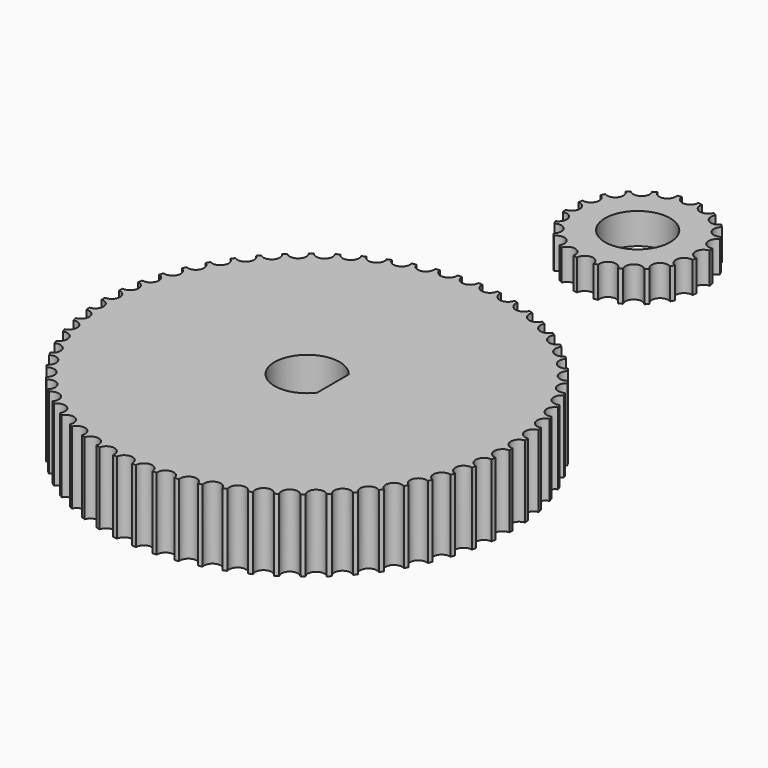
from build123d import *

# Parameters (mm, degrees)
F1_DEPTH = 3
F3_DEPTH = 7


with BuildPart() as f1:
    # F0 (on Top) → F1 (new body)
    with BuildSketch(Plane.XY):
        with BuildLine():
            ThreePointArc((6.3423941927, -0.7984322724), (5.5924532215, 0), (6.3423941927, 0.7984322724))
            ThreePointArc((6.3423941927, 0.7984322724), (6.3137515147, 1), (6.2787044669, 1.2005533751))
            ThreePointArc((6.2787044669, 1.2005533751), (5.3187390784, 1.7281630857), (5.7852461848, 2.7192618061))
            ThreePointArc((5.7852461848, 2.7192618061), (5.6957175259, 2.9021130326), (5.6004114016, 3.0820204934))
            ThreePointArc((5.6004114016, 3.0820204934), (4.5243896964, 3.2871615277), (4.6617979722, 4.3739110479))
            ThreePointArc((4.6617979722, 4.3739110479), (4.5201470213, 4.5201470213), (4.3739110479, 4.6617979722))
            ThreePointArc((4.3739110479, 4.6617979722), (3.2871615277, 4.5243896964), (3.0820204934, 5.6004114016))
            ThreePointArc((3.0820204934, 5.6004114016), (2.9021130326, 5.6957175259), (2.7192618061, 5.7852461848))
            ThreePointArc((2.7192618061, 5.7852461848), (1.7281630857, 5.3187390784), (1.2005533751, 6.2787044669))
            ThreePointArc((1.2005533751, 6.2787044669), (1, 6.3137515147), (0.7984322724, 6.3423941927))
            ThreePointArc((0.7984322724, 6.3423941927), (0, 5.5924532215), (-0.7984322724, 6.3423941927))
            ThreePointArc((-0.7984322724, 6.3423941927), (-1, 6.3137515147), (-1.2005533751, 6.2787044669))
            ThreePointArc((-1.2005533751, 6.2787044669), (-1.1816958118, 6.1799370569), (-1.1753766812, 6.0795842914))
            ThreePointArc((-1.1753766812, 6.0795842914), (-1.825556956, 5.2937382187), (-2.7192618061, 5.7852461848))
            ThreePointArc((-2.7192618061, 5.7852461848), (-2.9021130326, 5.6957175259), (-3.0820204934, 5.6004114016))
            ThreePointArc((-3.0820204934, 5.6004114016), (-2.9891790199, 5.3948795906), (-2.9573897296, 5.1716032919))
            ThreePointArc((-2.9573897296, 5.1716032919), (-3.4864811238, 4.418869257), (-4.3739110479, 4.6617979722))
            ThreePointArc((-4.3739110479, 4.6617979722), (-4.5201470213, 4.5201470213), (-4.6617979722, 4.3739110479))
            ThreePointArc((-4.6617979722, 4.3739110479), (-4.4477786392, 4.0980917579), (-4.3716032919, 3.7573897296))
            ThreePointArc((-4.3716032919, 3.7573897296), (-4.7862764746, 3.0563025425), (-5.6004114016, 3.0820204934))
            ThreePointArc((-5.6004114016, 3.0820204934), (-5.6957175259, 2.9021130326), (-5.7852461848, 2.7192618061))
            ThreePointArc((-5.7852461848, 2.7192618061), (-5.4179686608, 2.4251152245), (-5.2795842914, 1.9753766812))
            ThreePointArc((-5.2795842914, 1.9753766812), (-5.5893272876, 1.3431994353), (-6.2787044669, 1.2005533751))
            ThreePointArc((-6.2787044669, 1.2005533751), (-6.3137515147, 1), (-6.3423941927, 0.7984322724))
            ThreePointArc((-6.3423941927, 0.7984322724), (-5.8093377857, 0.5477010028), (-5.5924532215, 0))
            ThreePointArc((-5.5924532215, 0), (-5.8093377857, -0.5477010028), (-6.3423941927, -0.7984322724))
            ThreePointArc((-6.3423941927, -0.7984322724), (-6.3137515147, -1), (-6.2787044669, -1.2005533751))
            ThreePointArc((-6.2787044669, -1.2005533751), (-5.5893272876, -1.3431994353), (-5.2795842914, -1.9753766812))
            ThreePointArc((-5.2795842914, -1.9753766812), (-5.4179686608, -2.4251152245), (-5.7852461848, -2.7192618061))
            ThreePointArc((-5.7852461848, -2.7192618061), (-5.6957175259, -2.9021130326), (-5.6004114016, -3.0820204934))
            ThreePointArc((-5.6004114016, -3.0820204934), (-4.7862764746, -3.0563025425), (-4.3716032919, -3.7573897296))
            ThreePointArc((-4.3716032919, -3.7573897296), (-4.4477786392, -4.0980917579), (-4.6617979722, -4.3739110479))
            ThreePointArc((-4.6617979722, -4.3739110479), (-4.5201470213, -4.5201470213), (-4.3739110479, -4.6617979722))
            ThreePointArc((-4.3739110479, -4.6617979722), (-3.4864811238, -4.418869257), (-2.9573897296, -5.1716032919))
            ThreePointArc((-2.9573897296, -5.1716032919), (-2.9891790199, -5.3948795906), (-3.0820204934, -5.6004114016))
            ThreePointArc((-3.0820204934, -5.6004114016), (-2.9021130326, -5.6957175259), (-2.7192618061, -5.7852461848))
            ThreePointArc((-2.7192618061, -5.7852461848), (-1.825556956, -5.2937382187), (-1.1753766812, -6.0795842914))
            ThreePointArc((-1.1753766812, -6.0795842914), (-1.1816958118, -6.1799370569), (-1.2005533751, -6.2787044669))
            ThreePointArc((-1.2005533751, -6.2787044669), (-1, -6.3137515147), (-0.7984322724, -6.3423941927))
            ThreePointArc((-0.7984322724, -6.3423941927), (0, -5.5924532215), (0.7984322724, -6.3423941927))
            ThreePointArc((0.7984322724, -6.3423941927), (1, -6.3137515147), (1.2005533751, -6.2787044669))
            ThreePointArc((1.2005533751, -6.2787044669), (1.7281630857, -5.3187390784), (2.7192618061, -5.7852461848))
            ThreePointArc((2.7192618061, -5.7852461848), (2.9021130326, -5.6957175259), (3.0820204934, -5.6004114016))
            ThreePointArc((3.0820204934, -5.6004114016), (3.2871615277, -4.5243896964), (4.3739110479, -4.6617979722))
            ThreePointArc((4.3739110479, -4.6617979722), (4.5201470213, -4.5201470213), (4.6617979722, -4.3739110479))
            ThreePointArc((4.6617979722, -4.3739110479), (4.5243896964, -3.2871615277), (5.6004114016, -3.0820204934))
            ThreePointArc((5.6004114016, -3.0820204934), (5.6957175259, -2.9021130326), (5.7852461848, -2.7192618061))
            ThreePointArc((5.7852461848, -2.7192618061), (5.3187390784, -1.7281630857), (6.2787044669, -1.2005533751))
            ThreePointArc((6.2787044669, -1.2005533751), (6.3137515147, -1), (6.3423941927, -0.7984322724))
        make_face()
        with BuildLine():
            ThreePointArc((2.5, 1.9163767897), (2.9830772702, 1.0118053172), (3.15, 0))
            ThreePointArc((3.15, 0), (2.9830772702, -1.0118053172), (2.5, -1.9163767897))
            ThreePointArc((2.5, -1.9163767897), (-3.15, 0), (2.5, 1.9163767897))
        make_face(mode=Mode.SUBTRACT)
    extrude(amount=F1_DEPTH)


with BuildPart() as f3:
    # F2 (on Top) → F3 (new body)
    with BuildSketch(Plane.XY):
        with BuildLine():
            ThreePointArc((19.7426438555, -40.2003698738), (19.7434064237, -40.1001862267), (19.7436606153, -40))
            ThreePointArc((19.7436606153, -40), (19.7434064237, -39.8998137733), (19.7426438555, -39.7996301262))
            ThreePointArc((19.7426438555, -39.7996301262), (18.9193465628, -39.0405193351), (19.6616218184, -38.2020116903))
            ThreePointArc((19.6616218184, -38.2020116903), (19.6423622777, -38.0025669857), (19.6210796506, -37.8033280088))
            ThreePointArc((19.6210796506, -37.8033280088), (18.7252084651, -37.1314035752), (19.3788449351, -36.2221032999))
            ThreePointArc((19.3788449351, -36.2221032999), (19.3395067226, -36.025630337), (19.2981766169, -35.8295667186))
            ThreePointArc((19.2981766169, -35.8295667186), (18.3389243893, -35.2517234965), (18.8972148789, -34.280961242))
            ThreePointArc((18.8972148789, -34.280961242), (18.8382016581, -34.0894760993), (18.7772481765, -33.8985997173))
            ThreePointArc((18.7772481765, -33.8985997173), (17.7644581327, -33.4207671602), (18.221673826, -32.3985042609))
            ThreePointArc((18.221673826, -32.3985042609), (18.1435911524, -32.213971835), (18.0636397602, -32.0302413394))
            ThreePointArc((18.0636397602, -32.0302413394), (17.0077044965, -31.6573226559), (17.3591537418, -30.5940489125))
            ThreePointArc((17.3591537418, -30.5940489125), (17.2628028493, -30.4183627558), (17.1646739559, -30.2436634703))
            ThreePointArc((17.1646739559, -30.2436634703), (16.0764287971, -29.9794853106), (16.3185052495, -28.8861113505))
            ThreePointArc((16.3185052495, -28.8861113505), (16.2048748287, -28.7210742408), (16.0895753693, -28.5571988163))
            ThreePointArc((16.0895753693, -28.5571988163), (14.9801871834, -28.404472006), (15.110406811, -27.2922173256))
            ThreePointArc((15.110406811, -27.2922173256), (14.9806628636, -27.139522767), (14.8493759667, -26.9881527871))
            ThreePointArc((14.8493759667, -26.9881527871), (13.7302285777, -26.9484445098), (13.7472551508, -25.8287223473))
            ThreePointArc((13.7472551508, -25.8287223473), (13.6027290254, -25.6899371925), (13.4568018723, -25.5526259181))
            ThreePointArc((13.4568018723, -25.5526259181), (12.3393792469, -25.6263436346), (12.2430380499, -24.5106438545))
            ThreePointArc((12.2430380499, -24.5106438545), (12.08521278, -24.3871922271), (11.9261427807, -24.2653486576))
            ThreePointArc((11.9261427807, -24.2653486576), (10.8219111871, -24.4517359243), (10.613190811, -23.3515071162))
            ThreePointArc((10.613190811, -23.3515071162), (10.4436858976, -23.2446557969), (10.2731053255, -23.1395302123))
            ThreePointArc((10.2731053255, -23.1395302123), (9.1933956741, -23.4366744436), (8.8744378725, -22.3632064439))
            ThreePointArc((8.8744378725, -22.3632064439), (8.6949926653, -22.2740518718), (8.514651908, -22.1867230028))
            ThreePointArc((8.514651908, -22.1867230028), (7.4705434809, -22.5915750969), (7.0446211924, -21.5558831399))
            ThreePointArc((7.0446211924, -21.5558831399), (6.8570770421, -21.4853401616), (6.6688266397, -21.4167041206))
            ThreePointArc((6.6688266397, -21.4167041206), (5.6710334024, -21.925109747), (5.142517166, -20.9378214338))
            ThreePointArc((5.142517166, -20.9378214338), (4.9487985293, -20.8866139156), (4.7545701858, -20.8373750013))
            ThreePointArc((4.7545701858, -20.8373750013), (3.8133308469, -21.4441172304), (3.1876439545, -20.515363475))
            ThreePointArc((3.1876439545, -20.515363475), (2.9897386468, -20.4840168755), (2.7915254077, -20.4546803456))
            ThreePointArc((2.7915254077, -20.4546803456), (1.9164983568, -21.1535331811), (1.2000612024, -20.2928442538))
            ThreePointArc((1.2000612024, -20.2928442538), (1, -20.2816802315), (0.7998358015, -20.2725471187))
            ThreePointArc((0.7998358015, -20.2725471187), (0, -21.0563393847), (-0.7998358015, -20.2725471187))
            ThreePointArc((-0.7998358015, -20.2725471187), (-1, -20.2816802315), (-1.2000612024, -20.2928442538))
            ThreePointArc((-1.2000612024, -20.2928442538), (-1.1980903314, -20.3252143475), (-1.1974330143, -20.3576377223))
            ThreePointArc((-1.1974330143, -20.3576377223), (-1.9488218774, -21.1561594549), (-2.7915254077, -20.4546803456))
            ThreePointArc((-2.7915254077, -20.4546803456), (-2.9897386468, -20.4840168755), (-3.1876439545, -20.515363475))
            ThreePointArc((-3.1876439545, -20.515363475), (-3.1776951476, -20.5876254752), (-3.174369663, -20.6604932774))
            ThreePointArc((-3.174369663, -20.6604932774), (-3.885376456, -21.4555279993), (-4.7545701858, -20.8373750013))
            ThreePointArc((-4.7545701858, -20.8373750013), (-4.9487985293, -20.8866139156), (-5.142517166, -20.9378214338))
            ThreePointArc((-5.142517166, -20.9378214338), (-5.118562605, -21.048673163), (-5.1105239007, -21.1617983419))
            ThreePointArc((-5.1105239007, -21.1617983419), (-5.781377068, -21.9513052105), (-6.6688266397, -21.4167041206))
            ThreePointArc((-6.6688266397, -21.4167041206), (-6.8570770421, -21.4853401616), (-7.0446211924, -21.5558831399))
            ThreePointArc((-7.0446211924, -21.5558831399), (-7.0008130422, -21.7033166827), (-6.986028165, -21.8564088476))
            ThreePointArc((-6.986028165, -21.8564088476), (-7.6170592247, -22.63836121), (-8.514651908, -22.1867230028))
            ThreePointArc((-8.514651908, -22.1867230028), (-8.6949926653, -22.2740518718), (-8.8744378725, -22.3632064439))
            ThreePointArc((-8.8744378725, -22.3632064439), (-8.8051839303, -22.5445309851), (-8.7816372442, -22.7371971507))
            ThreePointArc((-8.7816372442, -22.7371971507), (-9.373279937, -23.5095877465), (-10.2731053255, -23.1395302123))
            ThreePointArc((-10.2731053255, -23.1395302123), (-10.4436858976, -23.2446557969), (-10.613190811, -23.3515071162))
            ThreePointArc((-10.613190811, -23.3515071162), (-10.5132273987, -23.5633795764), (-10.4789257592, -23.7951251713))
            ThreePointArc((-10.4789257592, -23.7951251713), (-11.0317149354, -24.555971285), (-11.9261427807, -24.2653486576))
            ThreePointArc((-11.9261427807, -24.2653486576), (-12.08521278, -24.3871922271), (-12.2430380499, -24.5106438545))
            ThreePointArc((-12.2430380499, -24.5106438545), (-12.1074993627, -24.7491069998), (-12.060477233, -25.0193371364))
            ThreePointArc((-12.060477233, -25.0193371364), (-12.5750474793, -25.7666856868), (-13.4568018723, -25.5526259181))
            ThreePointArc((-13.4568018723, -25.5526259181), (-13.6027290254, -25.6899371925), (-13.7472551508, -25.8287223473))
            ThreePointArc((-13.7472551508, -25.8287223473), (-13.5717383106, -26.0892499731), (-13.5100628075, -26.3972709746))
            ThreePointArc((-13.5100628075, -26.3972709746), (-13.9871468179, -27.1292035286), (-14.8493759667, -26.9881527871))
            ThreePointArc((-14.8493759667, -26.9881527871), (-14.9806628636, -27.139522767), (-15.110406811, -27.2922173256))
            ThreePointArc((-15.110406811, -27.2922173256), (-14.891031918, -27.5697660392), (-14.8128077729, -27.91478722))
            ThreePointArc((-14.8128077729, -27.91478722), (-15.2532344682, -28.6294249174), (-16.0895753693, -28.5571988163))
            ThreePointArc((-16.0895753693, -28.5571988163), (-16.2048748287, -28.7210742408), (-16.3185052495, -28.8861113505))
            ThreePointArc((-16.3185052495, -28.8861113505), (-16.0519697783, -29.1751784066), (-15.9553442031, -29.5563141024))
            ThreePointArc((-15.9553442031, -29.5563141024), (-16.3600366028, -30.2518224784), (-17.1646739559, -30.2436634703))
            ThreePointArc((-17.1646739559, -30.2436634703), (-17.2628028493, -30.4183627558), (-17.3591537418, -30.5940489125))
            ThreePointArc((-17.3591537418, -30.5940489125), (-17.0427806856, -30.8887354939), (-16.9259481282, -31.3050073347))
            ThreePointArc((-16.9259481282, -31.3050073347), (-17.2959209811, -31.9796010293), (-18.0636397602, -32.0302413394))
            ThreePointArc((-18.0636397602, -32.0302413394), (-18.1435911524, -32.213971835), (-18.221673826, -32.3985042609))
            ThreePointArc((-18.221673826, -32.3985042609), (-17.8534530591, -32.6925835359), (-17.7146598384, -33.1429229579))
            ThreePointArc((-17.7146598384, -33.1429229579), (-18.0510170182, -33.7948702988), (-18.7772481765, -33.8985997173))
            ThreePointArc((-18.7772481765, -33.8985997173), (-18.8382016581, -34.0894760993), (-18.8972148789, -34.280961242))
            ThreePointArc((-18.8972148789, -34.280961242), (-18.4758372767, -34.5679504823), (-18.3133860844, -35.0512014707))
            ThreePointArc((-18.3133860844, -35.0512014707), (-18.6173177554, -35.6788289184), (-19.2981766169, -35.8295667186))
            ThreePointArc((-19.2981766169, -35.8295667186), (-19.3395067226, -36.025630337), (-19.3788449351, -36.2221032999))
            ThreePointArc((-19.3788449351, -36.2221032999), (-18.9037288671, -36.4953392968), (-18.7159831245, -37.0102613532))
            ThreePointArc((-18.7159831245, -37.0102613532), (-18.9887626872, -37.611957797), (-19.6210796506, -37.8033280088))
            ThreePointArc((-19.6210796506, -37.8033280088), (-19.6423622777, -38.0025669857), (-19.6616218184, -38.2020116903))
            ThreePointArc((-19.6616218184, -38.2020116903), (-19.1329317092, -38.4547286731), (-18.9183197685, -39))
            ThreePointArc((-18.9183197685, -39), (-19.16130059, -39.5742208937), (-19.7426438555, -39.7996301262))
            ThreePointArc((-19.7426438555, -39.7996301262), (-19.7436606153, -40), (-19.7426438555, -40.2003698738))
            ThreePointArc((-19.7426438555, -40.2003698738), (-19.16130059, -40.4257791063), (-18.9183197685, -41))
            ThreePointArc((-18.9183197685, -41), (-19.1329317092, -41.5452713269), (-19.6616218184, -41.7979883097))
            ThreePointArc((-19.6616218184, -41.7979883097), (-19.6423622777, -41.9974330143), (-19.6210796506, -42.1966719912))
            ThreePointArc((-19.6210796506, -42.1966719912), (-18.9887626872, -42.388042203), (-18.7159831245, -42.9897386468))
            ThreePointArc((-18.7159831245, -42.9897386468), (-18.9037288671, -43.5046607032), (-19.3788449351, -43.7778967001))
            ThreePointArc((-19.3788449351, -43.7778967001), (-19.3395067226, -43.974369663), (-19.2981766169, -44.1704332814))
            ThreePointArc((-19.2981766169, -44.1704332814), (-18.6173177554, -44.3211710816), (-18.3133860844, -44.9487985293))
            ThreePointArc((-18.3133860844, -44.9487985293), (-18.4758372767, -45.4320495177), (-18.8972148789, -45.719038758))
            ThreePointArc((-18.8972148789, -45.719038758), (-18.8382016581, -45.9105239007), (-18.7772481765, -46.1014002827))
            ThreePointArc((-18.7772481765, -46.1014002827), (-18.0510170182, -46.2051297012), (-17.7146598384, -46.8570770421))
            ThreePointArc((-17.7146598384, -46.8570770421), (-17.8534530591, -47.3074164641), (-18.221673826, -47.6014957391))
            ThreePointArc((-18.221673826, -47.6014957391), (-18.1435911524, -47.786028165), (-18.0636397602, -47.9697586606))
            ThreePointArc((-18.0636397602, -47.9697586606), (-17.2959209811, -48.0203989707), (-16.9259481282, -48.6949926653))
            ThreePointArc((-16.9259481282, -48.6949926653), (-17.0427806856, -49.1112645061), (-17.3591537418, -49.4059510875))
            ThreePointArc((-17.3591537418, -49.4059510875), (-17.2628028493, -49.5816372442), (-17.1646739559, -49.7563365297))
            ThreePointArc((-17.1646739559, -49.7563365297), (-16.3600366028, -49.7481775216), (-15.9553442031, -50.4436858976))
            ThreePointArc((-15.9553442031, -50.4436858976), (-16.0519697783, -50.8248215934), (-16.3185052495, -51.1138886495))
            ThreePointArc((-16.3185052495, -51.1138886495), (-16.2048748287, -51.2789257592), (-16.0895753693, -51.4428011837))
            ThreePointArc((-16.0895753693, -51.4428011837), (-15.2532344682, -51.3705750826), (-14.8128077729, -52.08521278))
            ThreePointArc((-14.8128077729, -52.08521278), (-14.891031918, -52.4302339608), (-15.110406811, -52.7077826744))
            ThreePointArc((-15.110406811, -52.7077826744), (-14.9806628636, -52.860477233), (-14.8493759667, -53.0118472129))
            ThreePointArc((-14.8493759667, -53.0118472129), (-13.9871468179, -52.8707964714), (-13.5100628075, -53.6027290254))
            ThreePointArc((-13.5100628075, -53.6027290254), (-13.5717383106, -53.9107500269), (-13.7472551508, -54.1712776527))
            ThreePointArc((-13.7472551508, -54.1712776527), (-13.6027290254, -54.3100628075), (-13.4568018723, -54.4473740819))
            ThreePointArc((-13.4568018723, -54.4473740819), (-12.5750474793, -54.2333143132), (-12.060477233, -54.9806628636))
            ThreePointArc((-12.060477233, -54.9806628636), (-12.1074993627, -55.2508930002), (-12.2430380499, -55.4893561455))
            ThreePointArc((-12.2430380499, -55.4893561455), (-12.08521278, -55.6128077729), (-11.9261427807, -55.7346513424))
            ThreePointArc((-11.9261427807, -55.7346513424), (-11.0317149354, -55.444028715), (-10.4789257592, -56.2048748287))
            ThreePointArc((-10.4789257592, -56.2048748287), (-10.5132273987, -56.4366204236), (-10.613190811, -56.6484928838))
            ThreePointArc((-10.613190811, -56.6484928838), (-10.4436858976, -56.7553442031), (-10.2731053255, -56.8604697877))
            ThreePointArc((-10.2731053255, -56.8604697877), (-9.373279937, -56.4904122535), (-8.7816372442, -57.2628028493))
            ThreePointArc((-8.7816372442, -57.2628028493), (-8.8051839303, -57.4554690149), (-8.8744378725, -57.6367935561))
            ThreePointArc((-8.8744378725, -57.6367935561), (-8.6949926653, -57.7259481282), (-8.514651908, -57.8132769972))
            ThreePointArc((-8.514651908, -57.8132769972), (-7.6170592247, -57.36163879), (-6.986028165, -58.1435911524))
            ThreePointArc((-6.986028165, -58.1435911524), (-7.0008130422, -58.2966833173), (-7.0446211924, -58.4441168601))
            ThreePointArc((-7.0446211924, -58.4441168601), (-6.8570770421, -58.5146598384), (-6.6688266397, -58.5832958794))
            ThreePointArc((-6.6688266397, -58.5832958794), (-5.781377068, -58.0486947895), (-5.1105239007, -58.8382016581))
            ThreePointArc((-5.1105239007, -58.8382016581), (-5.118562605, -58.951326837), (-5.142517166, -59.0621785662))
            ThreePointArc((-5.142517166, -59.0621785662), (-4.9487985293, -59.1133860844), (-4.7545701858, -59.1626249987))
            ThreePointArc((-4.7545701858, -59.1626249987), (-3.885376456, -58.5444720007), (-3.174369663, -59.3395067226))
            ThreePointArc((-3.174369663, -59.3395067226), (-3.1776951476, -59.4123745248), (-3.1876439545, -59.484636525))
            ThreePointArc((-3.1876439545, -59.484636525), (-2.9897386468, -59.5159831245), (-2.7915254077, -59.5453196544))
            ThreePointArc((-2.7915254077, -59.5453196544), (-1.9488218774, -58.8438405451), (-1.1974330143, -59.6423622777))
            ThreePointArc((-1.1974330143, -59.6423622777), (-1.1980903314, -59.6747856525), (-1.2000612024, -59.7071557462))
            ThreePointArc((-1.2000612024, -59.7071557462), (-1, -59.7183197685), (-0.7998358015, -59.7274528813))
            ThreePointArc((-0.7998358015, -59.7274528813), (0, -58.9436606153), (0.7998358015, -59.7274528813))
            ThreePointArc((0.7998358015, -59.7274528813), (1, -59.7183197685), (1.2000612024, -59.7071557462))
            ThreePointArc((1.2000612024, -59.7071557462), (1.9164983568, -58.8464668189), (2.7915254077, -59.5453196544))
            ThreePointArc((2.7915254077, -59.5453196544), (2.9897386468, -59.5159831245), (3.1876439545, -59.484636525))
            ThreePointArc((3.1876439545, -59.484636525), (3.8133308469, -58.5558827696), (4.7545701858, -59.1626249987))
            ThreePointArc((4.7545701858, -59.1626249987), (4.9487985293, -59.1133860844), (5.142517166, -59.0621785662))
            ThreePointArc((5.142517166, -59.0621785662), (5.6710334024, -58.074890253), (6.6688266397, -58.5832958794))
            ThreePointArc((6.6688266397, -58.5832958794), (6.8570770421, -58.5146598384), (7.0446211924, -58.4441168601))
            ThreePointArc((7.0446211924, -58.4441168601), (7.4705434809, -57.4084249031), (8.514651908, -57.8132769972))
            ThreePointArc((8.514651908, -57.8132769972), (8.6949926653, -57.7259481282), (8.8744378725, -57.6367935561))
            ThreePointArc((8.8744378725, -57.6367935561), (9.1933956741, -56.5633255564), (10.2731053255, -56.8604697877))
            ThreePointArc((10.2731053255, -56.8604697877), (10.4436858976, -56.7553442031), (10.613190811, -56.6484928838))
            ThreePointArc((10.613190811, -56.6484928838), (10.8219111871, -55.5482640757), (11.9261427807, -55.7346513424))
            ThreePointArc((11.9261427807, -55.7346513424), (12.08521278, -55.6128077729), (12.2430380499, -55.4893561455))
            ThreePointArc((12.2430380499, -55.4893561455), (12.3393792469, -54.3736563654), (13.4568018723, -54.4473740819))
            ThreePointArc((13.4568018723, -54.4473740819), (13.6027290254, -54.3100628075), (13.7472551508, -54.1712776527))
            ThreePointArc((13.7472551508, -54.1712776527), (13.7302285777, -53.0515554902), (14.8493759667, -53.0118472129))
            ThreePointArc((14.8493759667, -53.0118472129), (14.9806628636, -52.860477233), (15.110406811, -52.7077826744))
            ThreePointArc((15.110406811, -52.7077826744), (14.9801871834, -51.595527994), (16.0895753693, -51.4428011837))
            ThreePointArc((16.0895753693, -51.4428011837), (16.2048748287, -51.2789257592), (16.3185052495, -51.1138886495))
            ThreePointArc((16.3185052495, -51.1138886495), (16.0764287971, -50.0205146894), (17.1646739559, -49.7563365297))
            ThreePointArc((17.1646739559, -49.7563365297), (17.2628028493, -49.5816372442), (17.3591537418, -49.4059510875))
            ThreePointArc((17.3591537418, -49.4059510875), (17.0077044965, -48.3426773441), (18.0636397602, -47.9697586606))
            ThreePointArc((18.0636397602, -47.9697586606), (18.1435911524, -47.786028165), (18.221673826, -47.6014957391))
            ThreePointArc((18.221673826, -47.6014957391), (17.7644581327, -46.5792328398), (18.7772481765, -46.1014002827))
            ThreePointArc((18.7772481765, -46.1014002827), (18.8382016581, -45.9105239007), (18.8972148789, -45.719038758))
            ThreePointArc((18.8972148789, -45.719038758), (18.3389243893, -44.7482765035), (19.2981766169, -44.1704332814))
            ThreePointArc((19.2981766169, -44.1704332814), (19.3395067226, -43.974369663), (19.3788449351, -43.7778967001))
            ThreePointArc((19.3788449351, -43.7778967001), (18.7252084651, -42.8685964248), (19.6210796506, -42.1966719912))
            ThreePointArc((19.6210796506, -42.1966719912), (19.6423622777, -41.9974330143), (19.6616218184, -41.7979883097))
            ThreePointArc((19.6616218184, -41.7979883097), (18.9193465628, -40.9594806649), (19.7426438555, -40.2003698738))
        make_face()
        with BuildLine():
            ThreePointArc((2.5, -38.0836232103), (2.9830772702, -38.9881946828), (3.15, -40))
            ThreePointArc((3.15, -40), (2.9830772702, -41.0118053172), (2.5, -41.9163767897))
            ThreePointArc((2.5, -41.9163767897), (-3.15, -40), (2.5, -38.0836232103))
        make_face(mode=Mode.SUBTRACT)
        with BuildLine():
            ThreePointArc((2.5, -41.9163767897), (2.9830772702, -41.0118053172), (3.15, -40))
            ThreePointArc((3.15, -40), (2.9830772702, -38.9881946828), (2.5, -38.0836232103))
            Line((2.5, -38.0836232103), (2.5, -41.9163767897))
        make_face()
    extrude(amount=F3_DEPTH)


solid = Compound([f1.part, f3.part])
